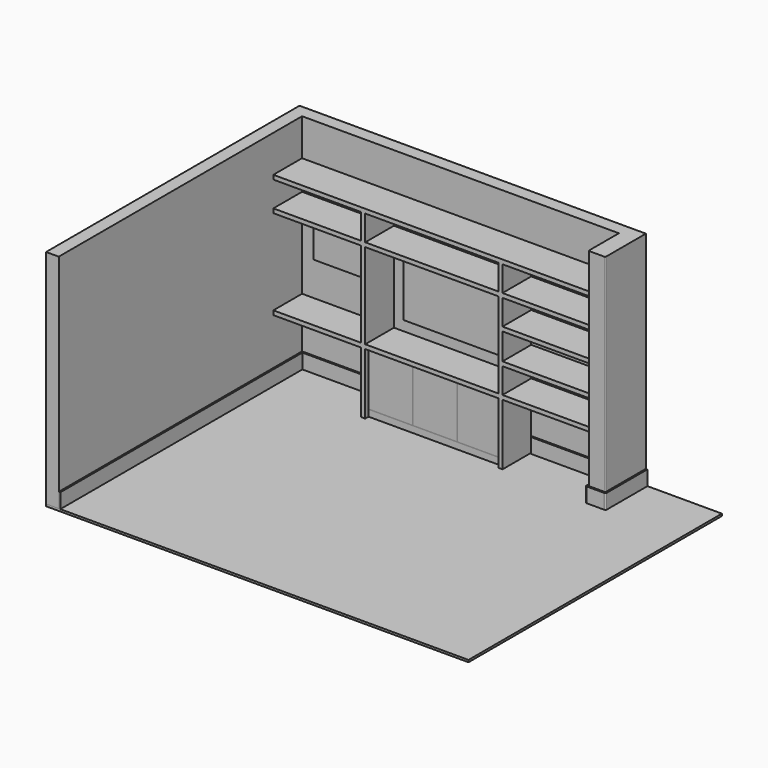
from build123d import *

# Parameters (mm, degrees)
F0_W      = 5080
F0_H      = 3810
F1_DEPTH  = 25.4
F3_DEPTH  = 2667
F4_W      = 3657.6
F4_H      = 177.8
F5_DEPTH  = 19.05
F7_W      = 438.15
F7_H      = 177.8
F8_DEPTH  = 19.05
F9_W      = 203.2
F9_H      = 177.8
F9_W_2    = 19.05
F10_DEPTH = 19.05
F11_W     = 609.6
F11_H     = 177.8
F11_W_2   = 19.05
F12_DEPTH = 19.05
F13_W     = 1346.2
F13_H     = 774.7
F14_DEPTH = 12.7
F15_W     = 1054.1
F15_H     = 50.8
F15_W_2   = 50.8
F15_W_3   = 1600.2
F15_H_2   = 1028.7
F15_H_3   = 736.6
F15_H_4   = 304.8
F16_DEPTH = 431.8
F17_W     = 381
F17_H     = 736.6
F18_DEPTH = 1600.2
F20_W     = 749.3
F20_H     = 457.2
F21_DEPTH = 19.05
F22_DEPTH = 19.05
F23_R     = 12.7
F23_2_R   = 12.7
F23_3_R   = 12.7
F24_W     = 1043.194326067
F24_H     = 177.8
F25_DEPTH = 19.05
F26_W     = 1043.6879966736
F26_H     = 177.8
F27_DEPTH = 19.05
F19_W     = 6.35
F19_H     = 654.05
F28_DEPTH = 6.35


# Not quite as in the source:
# - a feature names something its author has since deleted; it is built from what else it names


with BuildPart() as f1:
    # F0 (on Top) → F1 (new body)
    with BuildSketch(Plane.XY):
        Rectangle(F0_W, F0_H)
    extrude(amount=F1_DEPTH)

    # F4 (on face) → F5 (join)
    with BuildSketch(Plane.YZ.offset(-2387.6)):
        with Locations((-76.2, 114.3)):
            Rectangle(F4_W, F4_H)
    extrude(amount=F5_DEPTH)


with BuildPart() as f3:
    # F2 (on face) → F3 (new body)
    with BuildSketch(Plane.XY.offset(25.4)):
        Polygon((-2540, -1905), (-2387.6, -1905), (-2387.6, 1752.6), (1422.4, 1752.6), (1422.4, 1295.4), (1625.6, 1295.4), (1625.6, 1905), (-2540, 1905), align=None)
    extrude(amount=F3_DEPTH)

    # F23
    f23_edges = [f3.edges().sort_by_distance(p)[0] for p in [
        (1422.4, 1295.4, 1358.9),
        (1625.6, 1295.4, 1358.9),
    ]]
    fillet(f23_edges, radius=F23_R)


with BuildPart() as f8:
    # F7 (on face) → F8 (new body)
    with BuildSketch(Plane(origin=(1422.4, 0, 0), x_dir=(0, -1, 0), z_dir=(-1, 0, 0))):
        with Locations((-1514.475, 114.3)):
            Rectangle(F7_W, F7_H)
    extrude(amount=F8_DEPTH)


with BuildPart() as f10:
    # F9 (on face) → F10 (new body)
    with BuildSketch(Plane.XZ.offset(-1295.4)):
        with Locations((1524, 114.3)):
            Rectangle(F9_W, F9_H)
        with Locations((1412.875, 114.3)):
            Rectangle(F9_W_2, F9_H)
    extrude(amount=F10_DEPTH)

    # F23#2
    f23_2_edges = [f10.edges().sort_by_distance(p)[0] for p in [
        (1403.35, 1276.35, 114.3),
    ]]
    fillet(f23_2_edges, radius=F23_2_R)


with BuildPart() as f12:
    # F11 (on face) → F12 (new body)
    with BuildSketch(Plane.YZ.offset(1625.6)):
        with Locations((1600.2, 114.3)):
            Rectangle(F11_W, F11_H)
        with Locations((1285.875, 114.3)):
            Rectangle(F11_W_2, F11_H)
    extrude(amount=F12_DEPTH)

    # F23#3
    f23_3_edges = [f12.edges().sort_by_distance(p)[0] for p in [
        (1644.65, 1276.35, 114.3),
    ]]
    fillet(f23_3_edges, radius=F23_3_R)


with BuildPart() as f14:
    # F13 (on face) → F14 (new body)
    with BuildSketch(Plane.XZ.offset(-1752.6)):
        with Locations((-482.6, 1327.15)):
            Rectangle(F13_W, F13_H)
    extrude(amount=F14_DEPTH)


with BuildPart() as f16:
    # F15 (on face) → F16 (new body)
    with BuildSketch(Plane.XZ.offset(-1752.6)):
        Polygon((-2387.6, 2247.9), (-2387.6, 2197.1), (-1333.5, 2197.1), (-1282.7, 2197.1), (-1282.7, 2247.9), align=None)
        Polygon((-1282.7, 2247.9), (-1282.7, 2197.1), (317.5, 2197.1), (368.3, 2197.1), (1422.4, 2197.1), (1422.4, 2247.9), align=None)
        with Locations((-1860.55, 1866.9)):
            Rectangle(F15_W, F15_H)
        with Locations((-1308.1, 1866.9)):
            Rectangle(F15_W_2, F15_H)
        with Locations((-482.6, 1866.9)):
            Rectangle(F15_W_3, F15_H)
        with Locations((342.9, 1866.9)):
            Rectangle(F15_W_2, F15_H)
        with Locations((895.35, 1866.9)):
            Rectangle(F15_W, F15_H)
        with Locations((-1308.1, 1327.15)):
            Rectangle(F15_W_2, F15_H_2)
        Polygon((368.3, 1841.5), (317.5, 1841.5), (317.5, 812.8), (368.3, 812.8), (368.3, 1117.6), (368.3, 1168.4), (368.3, 1485.9), (368.3, 1536.7), align=None)
        with Locations((895.35, 787.4)):
            Rectangle(F15_W, F15_H)
        with Locations((342.9, 787.4)):
            Rectangle(F15_W_2, F15_H)
        with Locations((-482.6, 787.4)):
            Rectangle(F15_W_3, F15_H)
        with Locations((342.9, 393.7)):
            Rectangle(F15_W_2, F15_H_3)
        with Locations((-1308.1, 787.4)):
            Rectangle(F15_W_2, F15_H)
        with Locations((-1308.1, 393.7)):
            Rectangle(F15_W_2, F15_H_3)
        with Locations((-1860.55, 787.4)):
            Rectangle(F15_W, F15_H)
        with Locations((895.35, 1143)):
            Rectangle(F15_W, F15_H)
        with Locations((895.35, 1511.3)):
            Rectangle(F15_W, F15_H)
        with Locations((342.9, 2044.7)):
            Rectangle(F15_W_2, F15_H_4)
        with Locations((-1308.1, 2044.7)):
            Rectangle(F15_W_2, F15_H_4)
    extrude(amount=F16_DEPTH)


with BuildPart() as f18:
    # F17 (on face) → F18 (new body, through all)
    with BuildSketch(Plane.YZ.offset(-1282.7)):
        with Locations((1562.1, 393.7)):
            Rectangle(F17_W, F17_H)
    extrude(amount=F18_DEPTH)


with BuildPart() as f21:
    # F20 (on face) → F21 (new body)
    with BuildSketch(Plane.XZ.offset(-1752.6)):
        with Locations((-1860.55, 1460.5)):
            Rectangle(F20_W, F20_H)
    extrude(amount=F21_DEPTH)


with BuildPart() as f22:
    # F20 (on face) → F22 (new body)
    with BuildSketch(Plane.XZ.offset(-1752.6)):
        with Locations((-1860.55, 1460.5)):
            Rectangle(F20_W, F20_H)
    extrude(amount=F22_DEPTH)


with BuildPart() as f25:
    # F24 (on face) → F25 (new body)
    with BuildSketch(Plane.XZ.offset(-1752.6)):
        with Locations((900.8028369665, 114.3)):
            Rectangle(F24_W, F24_H)
    extrude(amount=F25_DEPTH)


with BuildPart() as f27:
    # F26 (on face) → F27 (new body)
    with BuildSketch(Plane.XZ.offset(-1752.6)):
        with Locations((-1846.7060016632, 114.3)):
            Rectangle(F26_W, F26_H)
    extrude(amount=F27_DEPTH)


with BuildPart() as f28:
    # F19 (on face) → F28 (new body)
    with BuildSketch(Plane.XZ.offset(-1371.6)):
        Polygon((-1282.7, 107.95), (-1282.7, 101.6), (317.5, 101.6), (317.5, 107.95), (-212.725, 107.95), (-219.075, 107.95), (-746.125, 107.95), (-752.475, 107.95), align=None)
        with Locations((-215.9, 434.975)):
            Rectangle(F19_W, F19_H)
        with Locations((-749.3, 434.975)):
            Rectangle(F19_W, F19_H)
    extrude(amount=-F28_DEPTH)


solid = Compound([f1.part, f3.part, f8.part, f10.part, f12.part, f14.part, f16.part, f18.part, f21.part, f22.part, f25.part, f27.part, f28.part])
